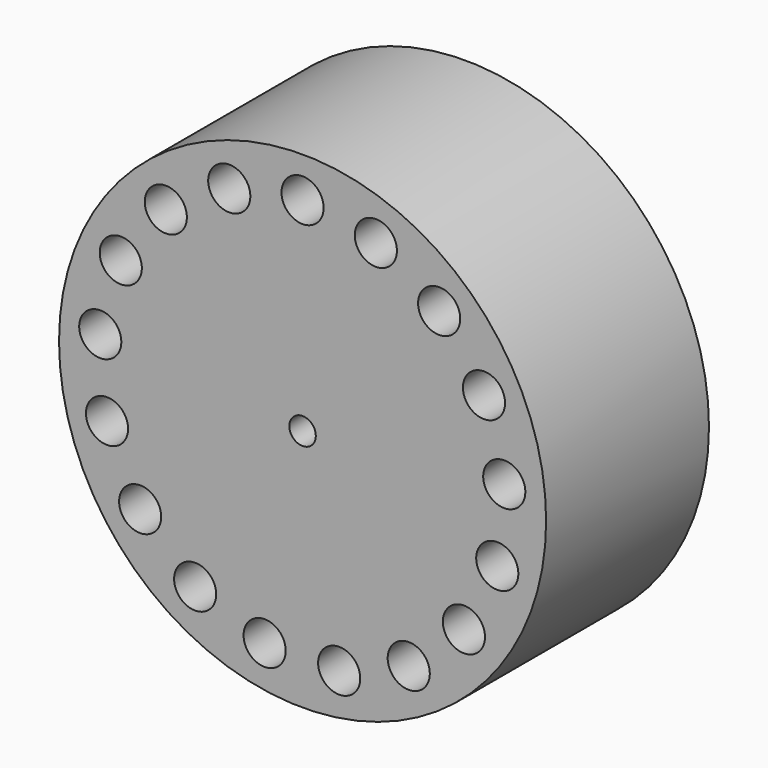
from build123d import *

# Parameters (mm, degrees)
F0_R     = 30.3902596551
F1_DEPTH = 25.4
F2_R     = 2.6289
F3_DEPTH = 35.306
F4_R     = 1.651
F5_DEPTH = 25.4


# Not quite as in the source:
# - a feature names something its author has since deleted; it is built from what else it names


with BuildPart() as f1:
    # F0 (on Front) → F1 (new body)
    with BuildSketch(Plane.XZ):
        Circle(F0_R)
    extrude(amount=F1_DEPTH)

    # F2 (on face) → F3 (cut)
    with BuildSketch(Plane.XZ.offset(25.4)):
        with Locations((-9.1471226763, 23.6621449357)):
            Circle(F2_R)
        with Locations((0, 25.3564708744)):
            Circle(F2_R)
        with Locations((-20.2673863665, -15.1786801491)):
            Circle(F2_R)
        with Locations((-24.4002614445, -6.8444173004)):
            Circle(F2_R)
        with Locations((-25.2433696844, 2.4200180379)):
            Circle(F2_R)
        with Locations((-22.6828446466, 11.3634125374)):
            Circle(F2_R)
        with Locations((-17.0644994257, 18.7779112138)):
            Circle(F2_R)
        with Locations((-4.7339240202, -24.8319767568)):
            Circle(F2_R)
        with Locations((-13.4029121308, -21.4571821289)):
            Circle(F2_R)
        with Locations((4.5687830844, -24.847279318)):
            Circle(F2_R)
        with Locations((9.1414989998, 23.6320609235)):
            Circle(F2_R)
        with Locations((17.0427642284, 18.721806202)):
            Circle(F2_R)
        with Locations((22.6366860342, 11.2888638188)):
            Circle(F2_R)
        with Locations((25.1677742804, 2.33709383)):
            Circle(F2_R)
        with Locations((24.294191474, -6.9245176239)):
            Circle(F2_R)
        with Locations((20.1339198139, -15.2451385957)):
            Circle(F2_R)
        with Locations((13.2488270404, -21.5010231169)):
            Circle(F2_R)
    extrude(amount=-F3_DEPTH, mode=Mode.SUBTRACT)

    # F4 (on face) → F5 (cut)
    with BuildSketch(Plane.XZ.offset(25.4)):
        Circle(F4_R)
    extrude(amount=-F5_DEPTH, mode=Mode.SUBTRACT)


solid = f1.part
